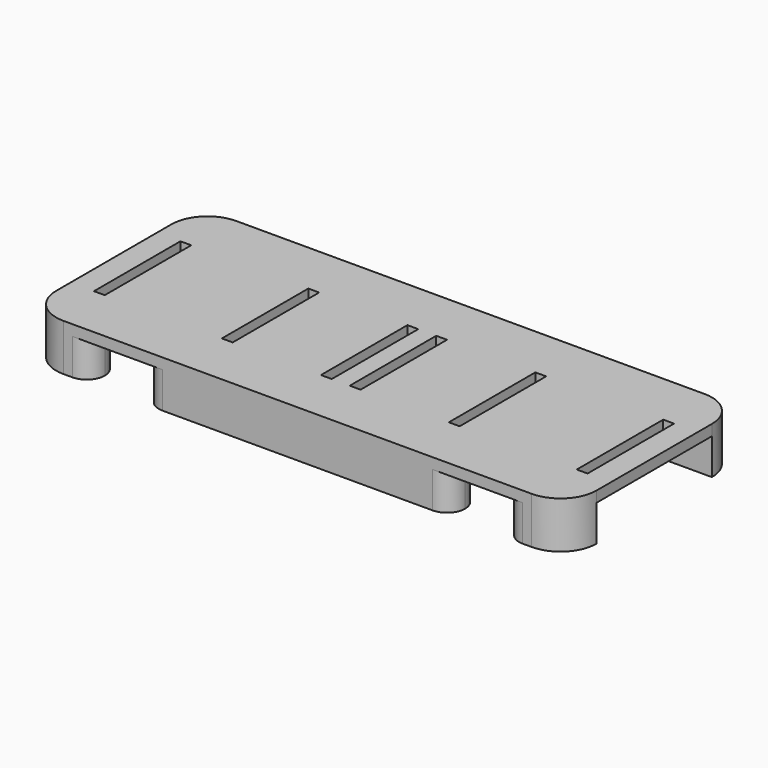
from build123d import *

# Parameters (mm, degrees)
F0_W     = 150
F0_H     = 60
F1_DEPTH = 3
F2_W     = 3
F2_H     = 30
F3_DEPTH = 25
F4_W     = 17.5
F4_H     = 10
F4_W_2   = 85
F5_DEPTH = 10
F6_R     = 10
F7_R     = 4.99999


# Not quite as in the source:
# - a fillet or chamfer is up to 0.001 mm smaller than in the source, because OpenCascade refuses the exact size


with BuildPart() as f1:
    # F0 (on Top) → F1 (new body)
    with BuildSketch(Plane.XY):
        Rectangle(F0_W, F0_H)
    extrude(amount=F1_DEPTH)

    # F2 (on Top) → F3 (cut)
    with BuildSketch(Plane.XY):
        with Locations((-67, 0)):
            Rectangle(F2_W, F2_H)
        with Locations((-31.5, 0)):
            Rectangle(F2_W, F2_H)
        with Locations((-4, 0)):
            Rectangle(F2_W, F2_H)
        with Locations((4, 0)):
            Rectangle(F2_W, F2_H)
        with Locations((31.5, 0)):
            Rectangle(F2_W, F2_H)
        with Locations((67, 0)):
            Rectangle(F2_W, F2_H)
    extrude(amount=F3_DEPTH, mode=Mode.SUBTRACT)

    # F4 (on Top) → F5 (join)
    with BuildSketch(Plane.XY):
        with Locations((-66.25, 25)):
            Rectangle(F4_W, F4_H)
        with Locations((66.25, 25)):
            Rectangle(F4_W, F4_H)
        with Locations((-66.25, -25)):
            Rectangle(F4_W, F4_H)
        with Locations((66.25, -25)):
            Rectangle(F4_W, F4_H)
        with Locations((0, 25)):
            Rectangle(F4_W_2, F4_H)
        with Locations((0, -25)):
            Rectangle(F4_W_2, F4_H)
    extrude(amount=-F5_DEPTH)

    # F6
    f6_edges = [f1.edges().sort_by_distance(p)[0] for p in [
        (-75, 30, -3.5),
        (-75, -30, -3.5),
        (75, -30, -3.5),
        (75, 30, -3.5),
    ]]
    fillet(f6_edges, radius=F6_R)

    # F7 (radius 5 in the source; OpenCascade refuses exactly that, so slightly less here)
    f7_edges = [f1.edges().sort_by_distance(p)[0] for p in [
        (57.5, 20, -5),
        (42.5, 20, -5),
        (57.5, -20, -5),
        (42.5, -20, -5),
        (42.5, -30, -5),
        (57.5, -30, -5),
        (57.5, 30, -5),
        (42.5, 30, -5),
        (-42.5, 20, -5),
        (-42.5, -30, -5),
        (-42.5, -20, -5),
        (-57.5, -20, -5),
        (-57.5, -30, -5),
        (-57.5, 20, -5),
        (-42.5, 30, -5),
        (-57.5, 30, -5),
    ]]
    fillet(f7_edges, radius=F7_R)


solid = f1.part
